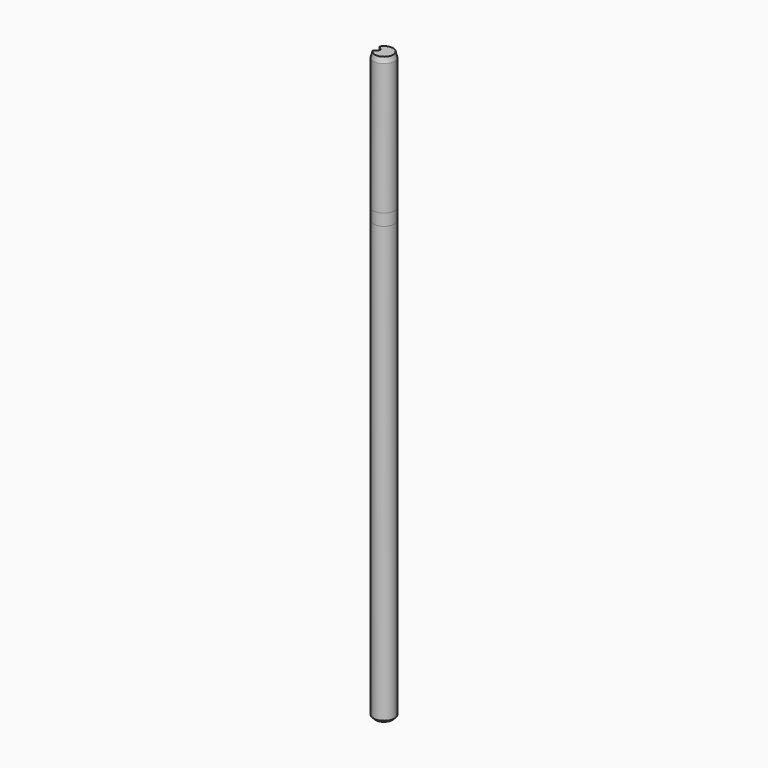
from build123d import *

# Parameters (mm, degrees)
F1_DEPTH  = 55
F2_SIZE2  = 0.2
F2_SIZE   = 0.2
F3_SIZE2  = 0.5
F3_SIZE   = 0.1339745962
F6_R      = 1.05
F6_R_2    = 0.8
F7_DEPTH  = 1.1
F9_R      = 1.05
F9_R_2    = 0.8
F10_DEPTH = 1.1
F13_R     = 1.05
F13_R_2   = 0.8
F14_DEPTH = 1.1
F16_R     = 1.05
F16_R_2   = 0.8
F17_DEPTH = 1.1
F19_R     = 0.9816666667
F19_R_2   = 0.8
F21_DEPTH = 1.1
F22_SCALE = 3


with BuildPart() as f1:
    # F0 (on Top) → F1 (new body)
    with BuildSketch(Plane.XY):
        with BuildLine():
            Line((-0.3890440115, -0.0707106781), (-0.8348150178, -0.5164816845))
            ThreePointArc((-0.8348150178, -0.5164816845), (0.9816666667, 0), (-0.8348150178, 0.5164816845))
            Line((-0.8348150178, 0.5164816845), (-0.3890440115, 0.0707106781))
            ThreePointArc((-0.3890440115, 0.0707106781), (-0.3597546896, 0), (-0.3890440115, -0.0707106781))
        make_face()
    extrude(amount=F1_DEPTH)

    # F2
    f2_edges = [f1.edges().sort_by_distance(p)[0] for p in [
        (0.981667, 0, 0),
    ]]
    chamfer(f2_edges, length=F2_SIZE, length2=F2_SIZE2)

    # F3
    f3_edges = [f1.edges().sort_by_distance(p)[0] for p in [
        (0.981667, 0, 55),
    ]]
    f3_side = f1.faces().sort_by_distance((0.100696, 0, 55))[0]
    chamfer(f3_edges, length=F3_SIZE, length2=F3_SIZE2, reference=f3_side)


with BuildPart() as f4_1:
    # F4: copy of F1
    add(f1.part)

    # F6 (on offset) → F7 (cut)
    with BuildSketch(Plane.XY.offset(36.15)):
        Circle(F6_R)
        Circle(F6_R_2, mode=Mode.SUBTRACT)
    extrude(amount=F7_DEPTH, mode=Mode.SUBTRACT)

    # F9 (on offset) → F10 (cut)
    with BuildSketch(Plane.XY.offset(41.65)):
        Circle(F9_R)
        Circle(F9_R_2, mode=Mode.SUBTRACT)
    extrude(amount=F10_DEPTH, mode=Mode.SUBTRACT)


with BuildPart() as f11_1:
    # F11: copy of F1
    add(f1.part)

    # F13 (on offset) → F14 (cut)
    with BuildSketch(Plane.XY.offset(22)):
        Circle(F13_R)
        Circle(F13_R_2, mode=Mode.SUBTRACT)
    extrude(amount=F14_DEPTH, mode=Mode.SUBTRACT)

    # F16 (on offset) → F17 (cut)
    with BuildSketch(Plane.XY.offset(27.5)):
        Circle(F16_R)
        Circle(F16_R_2, mode=Mode.SUBTRACT)
    extrude(amount=F17_DEPTH, mode=Mode.SUBTRACT)


with BuildPart() as f20_1:
    # F20: copy of F1
    add(f1.part)

    # F19 (on offset) → F21 (cut)
    with BuildSketch(Plane.XY.offset(41.05)):
        Circle(F19_R)
        Circle(F19_R_2, mode=Mode.SUBTRACT)
    extrude(amount=F21_DEPTH, mode=Mode.SUBTRACT)


with BuildPart() as f1_1:
    # F22: moved
    add(f1.part.scale(F22_SCALE))


with BuildPart() as f4_1_1:
    # F22: moved
    add(f4_1.part.scale(F22_SCALE))


with BuildPart() as f11_1_1:
    # F22: moved
    add(f11_1.part.scale(F22_SCALE))


with BuildPart() as f20_1_1:
    # F22: moved
    add(f20_1.part.scale(F22_SCALE))


solid = Compound([f1_1.part, f4_1_1.part, f11_1_1.part, f20_1_1.part])
